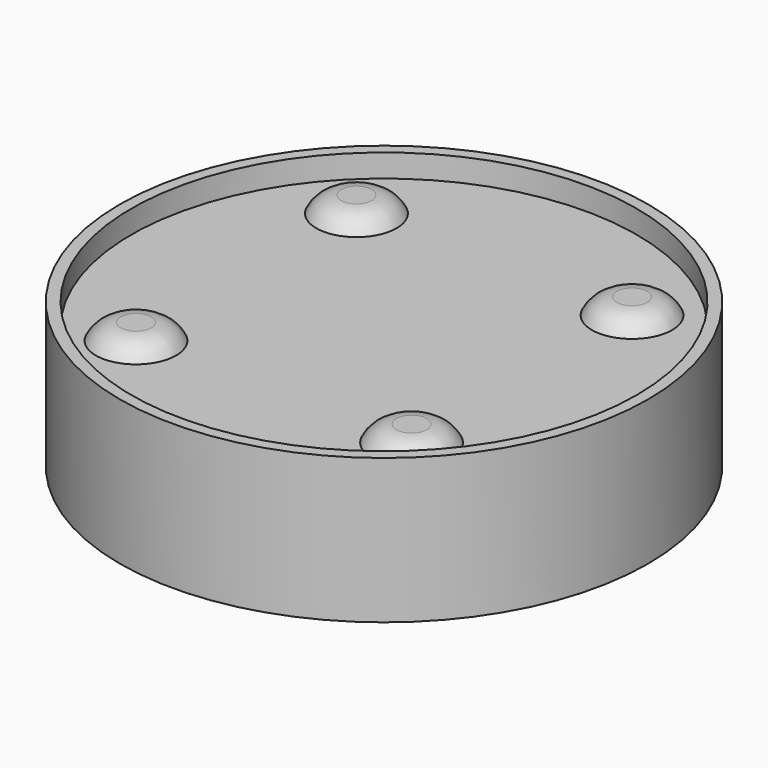
from build123d import *

# Parameters (mm, degrees)
F0_R           = 115
F1_DEPTH       = 15
F2_R           = 17.5
F3_DEPTH       = 38
F4_R           = 17.5
F5_DEPTH       = 7
F6_R           = 15.5
F7_DEPTH       = 15.5
F8_R           = 15.49999
F10_R          = 115
F10_R_2        = 110
F11_DEPTH      = 10
F11_DEPTH_BACK = 53


# Not quite as in the source:
# - a fillet or chamfer that OpenCascade refuses, or shapes differently, is made with other operations: its cross-section is extruded or revolved along the edge and cut away or added
# - a fillet or chamfer is up to 0.001 mm smaller than in the source, because OpenCascade refuses the exact size


with BuildPart() as f1:
    # F0 (on Top) → F1 (new body)
    with BuildSketch(Plane.XY):
        Circle(F0_R)
    extrude(amount=F1_DEPTH)

    # F2 (on face) → F3 (join)
    with BuildSketch(Plane(origin=(0, 0, 0), x_dir=(1, 0, 0), z_dir=(0, 0, -1))):
        Circle(F2_R)
    extrude(amount=F3_DEPTH)

    # F4 (on face) → F5 (join)
    with BuildSketch(Plane.XY.offset(15)):
        with Locations((-60, 60)):
            Circle(F4_R)
        with Locations((-60, -60)):
            Circle(F4_R)
        with Locations((60, -60)):
            Circle(F4_R)
        with Locations((60, 60)):
            Circle(F4_R)
    extrude(amount=F5_DEPTH)

    # F6 (on face) → F7 (cut)
    with BuildSketch(Plane(origin=(0, 0, 0), x_dir=(1, 0, 0), z_dir=(0, 0, -1))):
        with Locations((-60, 60)):
            Circle(F6_R)
        with Locations((-60, -60)):
            Circle(F6_R)
        with Locations((60, -60)):
            Circle(F6_R)
        with Locations((60, 60)):
            Circle(F6_R)
    extrude(amount=-F7_DEPTH, mode=Mode.SUBTRACT)

    # F8 (radius 15.5 in the source; OpenCascade refuses exactly that, so slightly less here)
    f8_edges = [f1.edges().sort_by_distance(p)[0] for p in [
        (-75.5, -60, 15.5),
        (44.5, -60, 15.5),
        (44.5, 60, 15.5),
        (-75.5, 60, 15.5),
    ]]
    fillet(f8_edges, radius=F8_R)

    # F9: fillet of radius 12 on 4 edges, made by hand

    # F9_s1 → F9_t2 (revolve, cut)
    with BuildSketch(Plane.XZ.offset(60)):
        with BuildLine():
            ThreePointArc((-42.5, 15), (-46.9279714162, 20.0995049384), (-53.4087121146, 22))
            Line((-53.4087121146, 22), (-42.5, 22))
            Line((-42.5, 22), (-42.5, 15))
        make_face()
    revolve(axis=Axis((-60, -60, 22), (0, 0, 1)), mode=Mode.SUBTRACT)

    # F9_s3 → F9_t4 (revolve, cut)
    with BuildSketch(Plane.XZ.offset(-60)):
        with BuildLine():
            ThreePointArc((-42.5, 15), (-46.9279714162, 20.0995049384), (-53.4087121146, 22))
            Line((-53.4087121146, 22), (-42.5, 22))
            Line((-42.5, 22), (-42.5, 15))
        make_face()
    revolve(axis=Axis((-60, 60, 22), (0, 0, 1)), mode=Mode.SUBTRACT)

    # F9_s5 → F9_t6 (revolve, cut)
    with BuildSketch(Plane.XZ.offset(-60)):
        with BuildLine():
            ThreePointArc((77.5, 15), (73.0720285838, 20.0995049384), (66.5912878854, 22))
            Line((66.5912878854, 22), (77.5, 22))
            Line((77.5, 22), (77.5, 15))
        make_face()
    revolve(axis=Axis((60, 60, 22), (0, 0, 1)), mode=Mode.SUBTRACT)

    # F9_s7 → F9_t8 (revolve, cut)
    with BuildSketch(Plane.XZ.offset(60)):
        with BuildLine():
            ThreePointArc((77.5, 15), (73.0720285838, 20.0995049384), (66.5912878854, 22))
            Line((66.5912878854, 22), (77.5, 22))
            Line((77.5, 22), (77.5, 15))
        make_face()
    revolve(axis=Axis((60, -60, 22), (0, 0, 1)), mode=Mode.SUBTRACT)

    # F10 (on face) → F11 (join, two sides)
    with BuildSketch(Plane.XY.offset(15)) as f11_sk:
        Circle(F10_R)
        Circle(F10_R_2, mode=Mode.SUBTRACT)
    extrude(amount=F11_DEPTH)
    extrude(f11_sk.sketch, amount=-F11_DEPTH_BACK)


solid = f1.part
